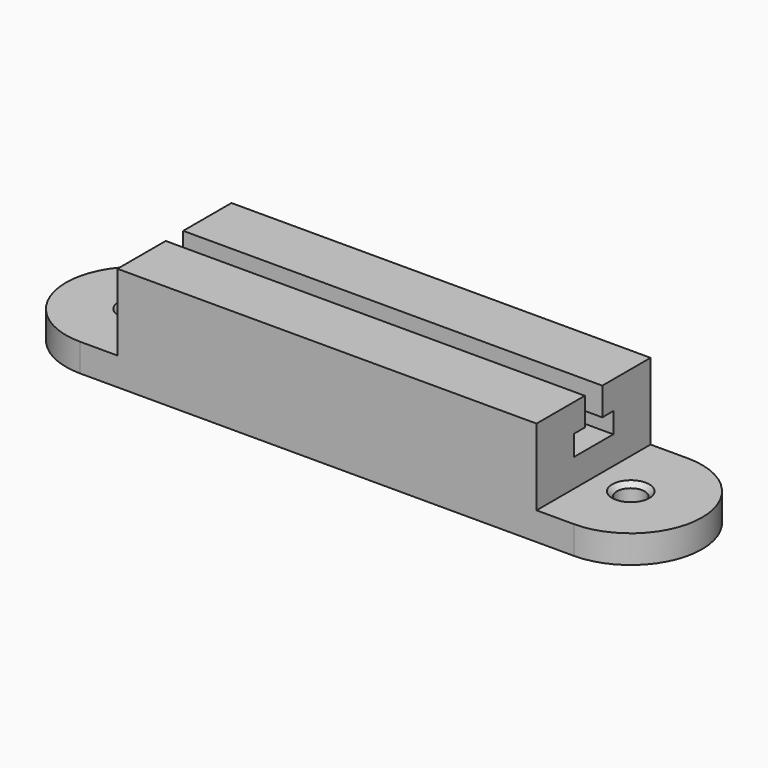
from build123d import *

# Parameters (mm, degrees)
F1_DEPTH       = 22.5
F2_W           = 45
F2_H           = 15.3
F3_DEPTH       = 3
F5_D           = 3
F5_DEPTH       = 4
F5_CSINK_D     = 4
F5_CSINK_ANGLE = 90
F5_TIP         = 0.9012909285


with BuildPart() as f1:
    # F0 (on Right) → F1 (new body, symmetric)
    with BuildSketch(Plane.YZ):
        Polygon((7.65, 0), (7.65, 11.2), (1.175, 11.2), (1.175, 8.2), (2.65, 8.2), (2.65, 6), (0, 6), (0, 0), align=None)
        Polygon((-7.65, 0), (0, 0), (0, 6), (-2.65, 6), (-2.65, 8.2), (-1.175, 8.2), (-1.175, 11.2), (-7.65, 11.2), align=None)
    extrude(amount=F1_DEPTH, both=True)

    # F2 (on face) → F3 (join)
    with BuildSketch(Plane(origin=(0, 0, 0), x_dir=(1, 0, 0), z_dir=(0, 0, -1))):
        with BuildLine():
            Line((22.5, 7.65), (22.5, -7.65))
            Line((22.5, -7.65), (26.5, -7.65))
            ThreePointArc((26.5, -7.65), (34.15, 0), (26.5, 7.65))
            Line((26.5, 7.65), (22.5, 7.65))
        make_face()
        Rectangle(F2_W, F2_H)
        with BuildLine():
            Line((-26.5, -7.65), (-22.5, -7.65))
            Line((-22.5, -7.65), (-22.5, 7.65))
            Line((-22.5, 7.65), (-26.5, 7.65))
            ThreePointArc((-26.5, 7.65), (-34.15, 0), (-26.5, -7.65))
        make_face()
    extrude(amount=-F3_DEPTH)

    # F5
    with Locations(Plane.XY.offset(3)):
        with Locations((26.5, 0), (-26.5, 0)):
            CounterSinkHole(F5_D / 2, F5_CSINK_D / 2, depth=F5_DEPTH, counter_sink_angle=F5_CSINK_ANGLE)
            with Locations((0, 0, -(F5_DEPTH + F5_TIP / 2))):  # 118° drill point
                Cone(0, F5_D / 2, F5_TIP, mode=Mode.SUBTRACT)


solid = f1.part
